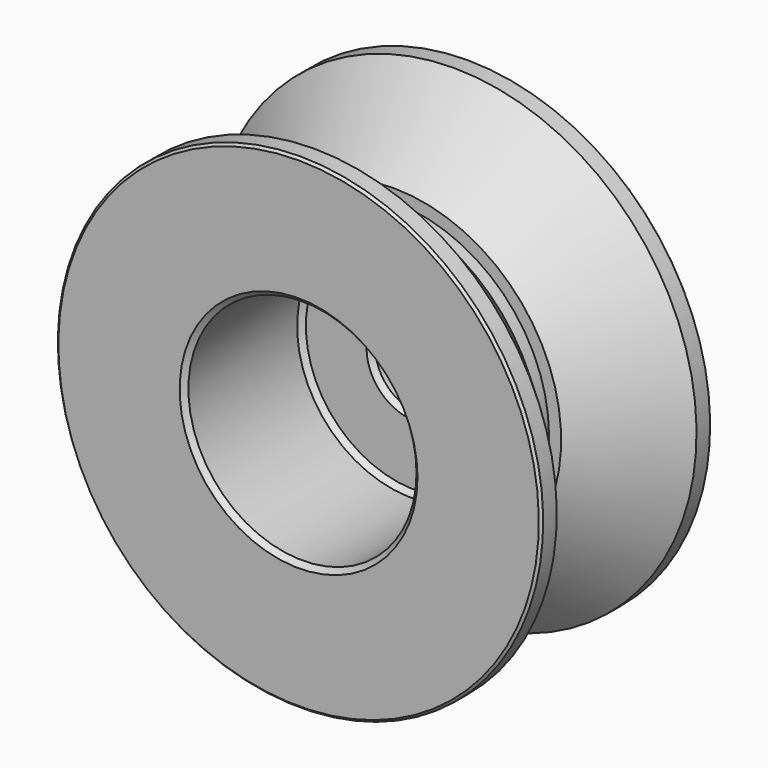
from build123d import *

# Parameters (mm, degrees)
F2_SIZE  = 0.5
F3_R     = 23.5
F4_DEPTH = 30
F5_SIZE  = 1


with BuildPart() as f1:
    # F0 (on Right) → F1 (revolve)
    with BuildSketch(Plane.YZ):
        Polygon((-40.5099816322, 9), (3.4900183678, 9), (3.4900183678, 50), (-0.5099816322, 50), (-16.0099816322, 34.5), (-16.0099816322, 32), (-21.0099816322, 32), (-21.0099816322, 34.5), (-36.5099816322, 50), (-40.5099816322, 50), align=None)
    revolve(axis=Axis((0, -20.3511445433, 0), (0, 1, 0)))

    # F2
    f2_edges = [f1.edges().sort_by_distance(p)[0] for p in [
        (0, -40.509982, -9),
        (0, -40.509982, -50),
        (0, 3.490018, -50),
        (0, 3.490018, -9),
    ]]
    chamfer(f2_edges, length=F2_SIZE)

    # F3 (on face) → F4 (cut)
    with BuildSketch(Plane.XZ.offset(40.5099816322)):
        Circle(F3_R)
    extrude(amount=-F4_DEPTH, mode=Mode.SUBTRACT)

    # F5
    f5_edges = [f1.edges().sort_by_distance(p)[0] for p in [
        (-23.5, -40.509982, 0),
        (0, -10.509982, -9),
        (-23.5, -10.509982, 0),
    ]]
    chamfer(f5_edges, length=F5_SIZE)


solid = f1.part
